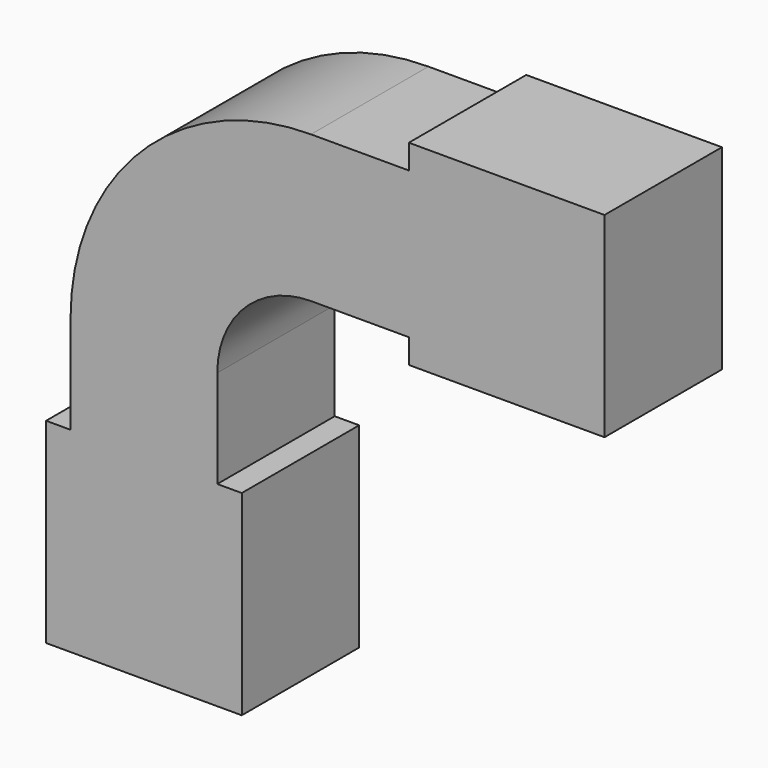
from build123d import *

# Parameters (mm, degrees)
F1_DEPTH = 19.05


# Not quite as in the source:
# - a feature of the source that left no trace in its solid (it failed there, or was rolled back) is left out


with BuildPart() as f1:
    # F0 (on Front) → F1 (new body, symmetric)
    with BuildSketch(Plane.XZ):
        with BuildLine():
            Line((-19.05, 50.8), (-19.05, 25.4))
            Line((-19.05, 25.4), (19.05, 25.4))
            Line((19.05, 25.4), (19.05, 50.8))
            ThreePointArc((19.05, 50.8), (26.174342016, 67.9996831179), (43.3740251338, 75.1240251338))
            Line((43.3740251338, 75.1240251338), (68.7740251338, 75.1240251338))
            Line((68.7740251338, 75.1240251338), (68.7740251338, 113.2240251338))
            Line((68.7740251338, 113.2240251338), (43.3740251338, 113.2240251338))
            ThreePointArc((43.3740251338, 113.2240251338), (-0.7664263473, 94.9404514811), (-19.05, 50.8))
        make_face()
        Polygon((-19.05, 25.4), (-25.4, 25.4), (-25.4, -25.4), (25.4, -25.4), (25.4, 25.4), (19.05, 25.4), align=None)
        Polygon((68.7740251338, 119.5740251338), (68.7740251338, 113.2240251338), (68.7740251338, 75.1240251338), (68.7740251338, 68.7740251338), (119.5740251338, 68.7740251338), (119.5740251338, 119.5740251338), align=None)
    extrude(amount=F1_DEPTH, both=True)


solid = f1.part
